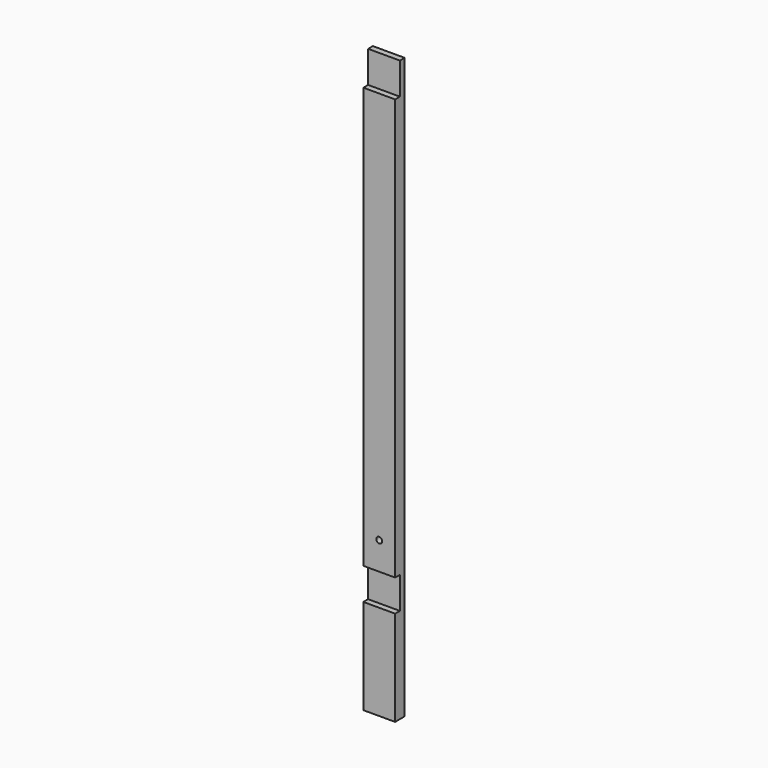
from build123d import *

# Parameters (mm, degrees)
F0_W     = 50.8
F0_H     = 19.05
F1_DEPTH = 927.1
F2_W     = 122.43557321
F2_H     = 50.8
F2_W_2   = 343.1604206562
F3_DEPTH = 25.4
F4_R     = 4.7625
F5_DEPTH = 25.4


# Not quite as in the source:
# - a feature names something its author has since deleted; it is built from what else it names


with BuildPart() as f1:
    # F0 (on Top) → F1 (new body)
    with BuildSketch(Plane.XY):
        Rectangle(F0_W, F0_H)
    extrude(amount=F1_DEPTH)

    # F2 (on Front) → F3 (cut)
    with BuildSketch(Plane.XZ):
        with Locations((22.4465244144, 177.8)):
            Rectangle(F2_W, F2_H)
        with Locations((-38.7818217278, 901.7)):
            Rectangle(F2_W_2, F2_H)
    extrude(amount=F3_DEPTH, mode=Mode.SUBTRACT)

    # F4 (on Front) → F5 (cut)
    with BuildSketch(Plane.XZ):
        with Locations((0, 247.65)):
            Circle(F4_R)
    extrude(amount=F5_DEPTH, mode=Mode.SUBTRACT)


solid = f1.part
